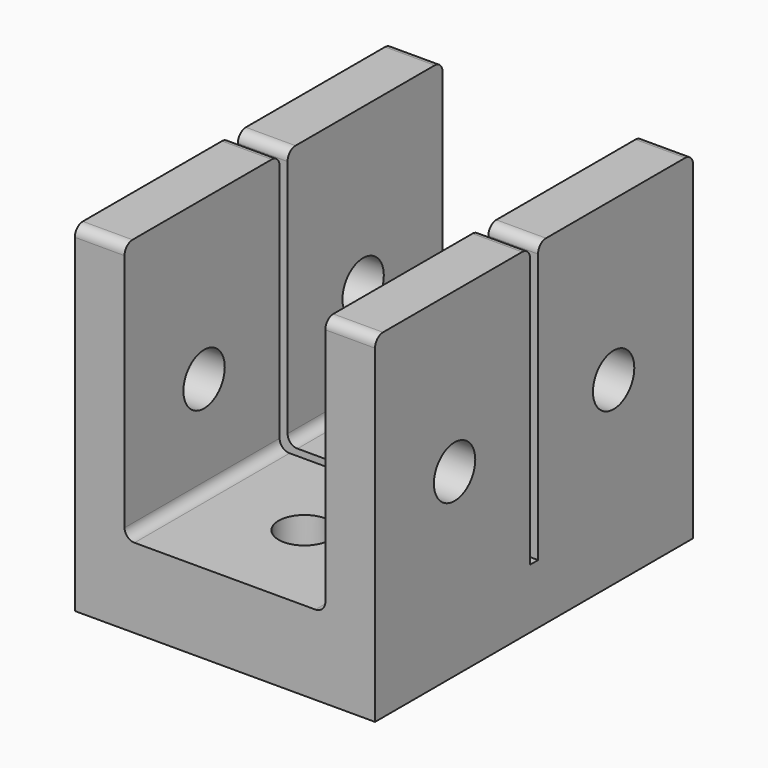
from build123d import *

# Parameters (mm, degrees)
F2_DEPTH      = 20
F3_W          = 1
F3_H          = 28.1
F4_DEPTH      = 15.101
F4_DEPTH_BACK = 15.101
F5_R          = 2.6
F6_DEPTH      = 15.101
F6_DEPTH_BACK = 15.101
F7_R          = 2.6
F8_DEPTH      = 8
F9_R          = 5
F10_DEPTH     = 3
F11_S5_R      = 5
F11_T6_DEPTH  = 9
F11_S11_R     = 5
F11_T12_DEPTH = 9
F12_R         = 1


# Not quite as in the source:
# - a fillet or chamfer that OpenCascade refuses, or shapes differently, is made with other operations: its cross-section is extruded or revolved along the edge and cut away or added


with BuildPart() as f2:
    # F1 (on Front) → F2 (new body, symmetric)
    with BuildSketch(Plane.XZ):
        Polygon((15.1, 16), (10.1, 16), (10.1, -10.1), (-10.1, -10.1), (-10.1, 16), (-15.1, 16), (-15.1, -18.1), (15.1, -18.1), align=None)
    extrude(amount=F2_DEPTH, both=True)

    # F3 (on Right) → F4 (cut, two sides)
    with BuildSketch(Plane.YZ) as f4_sk:
        with Locations((0, 1.95)):
            Rectangle(F3_W, F3_H)
    extrude(amount=-F4_DEPTH, mode=Mode.SUBTRACT)
    extrude(f4_sk.sketch, amount=F4_DEPTH_BACK, mode=Mode.SUBTRACT)

    # F5 (on Right) → F6 (cut, two sides)
    with BuildSketch(Plane.YZ) as f6_sk:
        with Locations((10, 0)):
            Circle(F5_R)
        with Locations((-10, 0)):
            Circle(F5_R)
    extrude(amount=-F6_DEPTH, mode=Mode.SUBTRACT)
    extrude(f6_sk.sketch, amount=F6_DEPTH_BACK, mode=Mode.SUBTRACT)

    # F7 (on face) → F8 (cut, through all)
    with BuildSketch(Plane(origin=(0, 0, -18.1), x_dir=(1, 0, 0), z_dir=(0, 0, -1))):
        with Locations((0, 10)):
            Circle(F7_R)
        with Locations((0, -10)):
            Circle(F7_R)
    extrude(amount=-F8_DEPTH, mode=Mode.SUBTRACT)

    # F9 (on face) → F10 (cut)
    with BuildSketch(Plane(origin=(0, 0, -18.1), x_dir=(1, 0, 0), z_dir=(0, 0, -1))):
        with Locations((0, 10)):
            Circle(F9_R)
        with Locations((0, -10)):
            Circle(F9_R)
    extrude(amount=-F10_DEPTH, mode=Mode.SUBTRACT)

    # F11: chamfer of 2.5 x 1.443375673 on 2 edges, made by hand


with BuildPart() as f11_tool2:
    # F11_s3 → F11_t4 (revolve)
    with BuildSketch(Plane.XZ.offset(10)):
        Polygon((5.1, -15.1), (2.6, -13.656624327), (2.6, -15.1), align=None)
    revolve(axis=Axis((0, -10, -15.1), (0, 0, -1)))

    # F11_s5 → F11_t6 (intersect, symmetric)
    with BuildSketch(Plane.XY.offset(-14.4)):
        with Locations((0, -10)):
            Circle(F11_S5_R)
    extrude(amount=F11_T6_DEPTH, both=True, mode=Mode.INTERSECT)


with BuildPart() as f2_1:
    add(f2.part)

    # F11_t1: cut F11_tool2
    add(f11_tool2.part, mode=Mode.SUBTRACT)


with BuildPart() as f11_tool8:
    # F11_s9 → F11_t10 (revolve)
    with BuildSketch(Plane.XZ.offset(-10)):
        Polygon((2.6, -13.656624327), (5.1, -15.1), (2.6, -15.1), align=None)
    revolve(axis=Axis((0, 10, -15.1), (0, 0, -1)))

    # F11_s11 → F11_t12 (intersect, symmetric)
    with BuildSketch(Plane.XY.offset(-14.4)):
        with Locations((0, 10)):
            Circle(F11_S11_R)
    extrude(amount=F11_T12_DEPTH, both=True, mode=Mode.INTERSECT)


with BuildPart() as f2_2:
    add(f2_1.part)

    # F11_t7: cut F11_tool8
    add(f11_tool8.part, mode=Mode.SUBTRACT)

    # F12
    f12_edges = [f2_2.edges().sort_by_distance(p)[0] for p in [
        (-10.1, -10.25, -10.1),
        (-10.1, 10.25, -10.1),
        (10.1, -10.25, -10.1),
        (10.1, 10.25, -10.1),
        (-12.6, 20, 16),
        (12.6, 0.5, 16),
        (-12.6, 0.5, 16),
        (12.6, -0.5, 16),
        (-12.6, -0.5, 16),
        (-12.6, -20, 16),
        (12.6, 20, 16),
        (12.6, -20, 16),
    ]]
    fillet(f12_edges, radius=F12_R)


solid = f2_2.part
